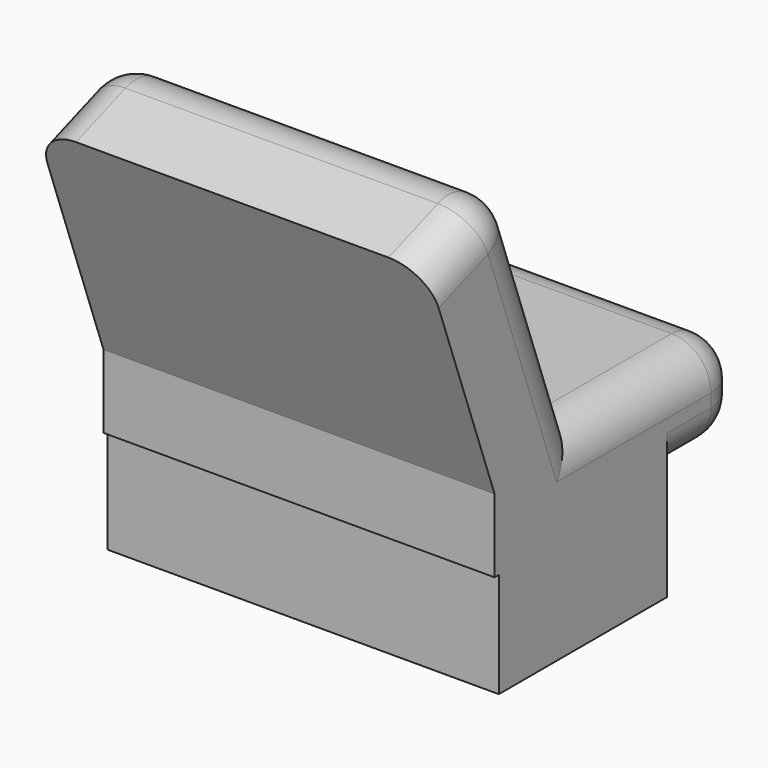
from build123d import *

# Parameters (mm, degrees)
F0_W        = 7.45
F0_H        = 4
F1_DEPTH    = 2
F2_W        = 7.45
F2_H        = 5.9
F3_DEPTH    = 1.75
F6_W        = 7.45
F6_H        = 5
F7_DEPTH    = 2
F8_R        = 0.75
F9_T1_DEPTH = 1.05
F9_S5_W     = 0.75
F9_S5_H     = 0.75
F9_T6_DEPTH = 0.75


# Not quite as in the source:
# - a fillet or chamfer that OpenCascade refuses, or shapes differently, is made with other operations: its cross-section is extruded or revolved along the edge and cut away or added


with BuildPart() as f1:
    # F0 (on Top) → F1 (new body)
    with BuildSketch(Plane.XY):
        with Locations((3.725, 2)):
            Rectangle(F0_W, F0_H)
    extrude(amount=F1_DEPTH)

    # F2 (on face) → F3 (join)
    with BuildSketch(Plane.XY.offset(2)):
        with Locations((3.725, 2.85)):
            Rectangle(F2_W, F2_H)
    extrude(amount=F3_DEPTH)

    # F6 (on line) → F7 (join)
    with BuildSketch(Plane(origin=(0, 2.8829689891, 1.0493148984), x_dir=(-1, 0, 0), z_dir=(0, 0.9396926208, 0.3420201433))):
        with Locations((-3.725, 5.3740090556)):
            Rectangle(F6_W, F6_H)
    extrude(amount=-F7_DEPTH)

    # F8
    f8_edges = [f1.edges().sort_by_distance(p)[0] for p in [
        (7.45, 5.8, 2.875),
        (7.45, 3.85, 3.75),
        (3.725, 5.8, 3.75),
        (3.725, 5.8, 2),
        (0, 5.8, 2.875),
        (0, 3.85, 3.75),
        (0, 4.9, 2),
        (0, 1.04495, 6.099232),
        (3.725, 0.189899, 8.448463),
        (7.45, 1.04495, 6.099232),
        (7.45, -0.749793, 8.106443),
        (0, -0.749793, 8.106443),
    ]]
    fillet(f8_edges, radius=F8_R)

    # F9: fillet of radius 0.75 on 1 edges, made by hand

    # F9_s2 → F9_t1 (cut)
    with BuildSketch(Plane.XZ.offset(-5.05)):
        with BuildLine():
            ThreePointArc((7.45, 2.75), (7.2303300859, 2.2196699141), (6.7, 2))
            Line((6.7, 2), (7.45, 2))
            Line((7.45, 2), (7.45, 2.75))
        make_face()
    extrude(amount=F9_T1_DEPTH, mode=Mode.SUBTRACT)


with BuildPart() as f9_tool4:
    # F9_s5 → F9_t6 (new body)
    with BuildSketch(Plane.YZ.offset(6.7)):
        with Locations((5.425, 2.375)):
            Rectangle(F9_S5_W, F9_S5_H)
    extrude(amount=F9_T6_DEPTH)

    # F9_s7 → F9_t8 (revolve, cut)
    with BuildSketch(Plane(origin=(6.7, 5.05, 2.75), x_dir=(0, -0.7071067812, 0.7071067812), z_dir=(0, 0.7071067812, 0.7071067812))):
        with BuildLine():
            ThreePointArc((0, -0.75), (0.75, 0), (0, 0.75))
            Line((0, 0.75), (0, -0.75))
        make_face()
    revolve(axis=Axis((6.7, 5.05, 2.75), (1, 0, 0)), mode=Mode.SUBTRACT)


with BuildPart() as f1_1:
    add(f1.part)

    # F9_t3: cut F9_tool4
    add(f9_tool4.part, mode=Mode.SUBTRACT)


solid = f1_1.part
